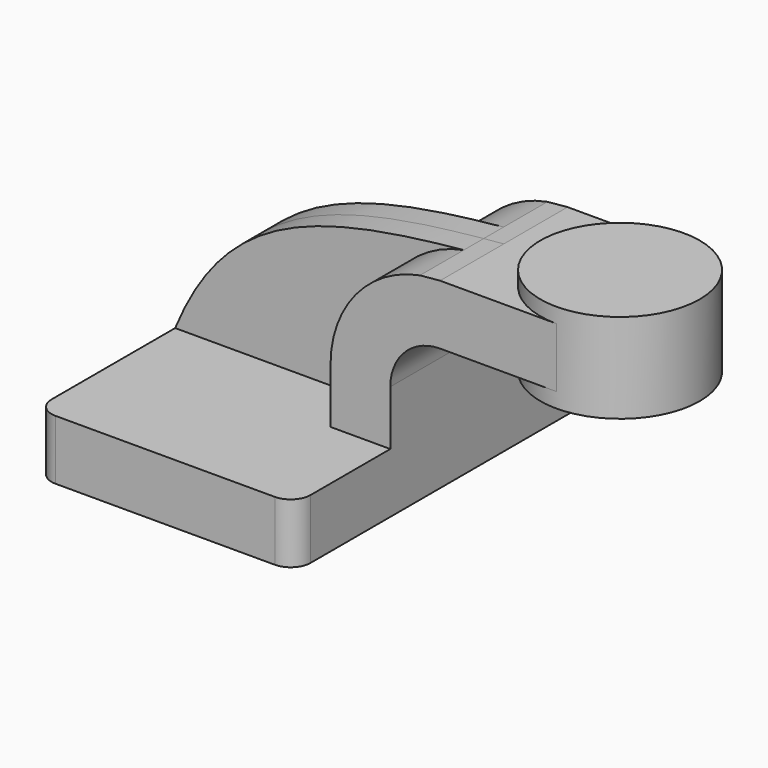
from build123d import *

# Parameters (mm, degrees)
F1_DEPTH = 63.5
F2_DEPTH = 25.4
F3_DEPTH = 7.9375
F0_W     = 25.4
F0_H     = 19.05
F4_DEPTH = 25.4
F6_R     = 6.35


# Not quite as in the source:
# - ends of sketch curves that miss each other by under 0.0002 mm in the source are joined
# - a feature names something its author has since deleted; it is built from what else it names


with BuildPart() as f1:
    # F0 (on Front) → F1 (new body, symmetric)
    with BuildSketch(Plane.XZ):
        Polygon((41.275, -9.525), (41.275, 9.525), (22.225, 9.525), (-41.275, 9.525), (-41.275, -9.525), align=None)
    extrude(amount=F1_DEPTH, both=True)

    # F0 (on Front) → F2 (join, symmetric)
    with BuildSketch(Plane.XZ):
        with BuildLine():
            Line((22.225, 9.525), (41.275, 9.525))
            Line((41.275, 9.525), (41.275, 27.0002))
            ThreePointArc((41.275, 27.0002), (45.9246798487, 38.2255201513), (57.15, 42.8752))
            Line((57.15, 42.8752), (68.7916731741, 42.8752))
            Line((68.7916731741, 42.8752), (68.7916731741, 61.9252))
            Line((68.7916731741, 61.9252), (57.15, 61.9252))
            add(Edge.make_bspline(
                [(50.7252492869, 61.329171511), (52.8269652502, 61.534305037), (54.9682888804, 61.732284225), (57.15, 61.9252)],
                knots=[106.8911851376, 106.8911851376, 106.8911851376, 106.8911851376, 111.5045367133, 111.5045367133, 111.5045367133, 111.5045367133], degree=3))
            ThreePointArc((50.7252492869, 61.329171511), (30.2786385449, 49.3090690945), (22.22499883, 27.0002))
            Line((22.22499883, 27.0002), (22.225, 9.525))
        make_face()
    extrude(amount=F2_DEPTH, both=True)

    # F0 (on Front) → F3 (join, symmetric)
    with BuildSketch(Plane.XZ):
        with BuildLine():
            Line((-41.275, 9.525), (22.225, 9.525))
            Line((22.225, 9.525), (22.225, 27.0002))
            ThreePointArc((22.225, 27.0002), (30.2786385449, 49.3090690945), (50.7252492869, 61.329171511))
            add(Edge.make_bspline(
                [(-41.275, 9.525), (-25.4048483065, 47.9825129098), (2.0285682627, 56.5762353117), (50.7252492869, 61.329171511)],
                knots=[0, 0, 0, 0, 106.8911851376, 106.8911851376, 106.8911851376, 106.8911851376], degree=3))
        make_face()
    extrude(amount=F3_DEPTH, both=True)

    # F0 (on Front) → F4 (join, symmetric)
    with BuildSketch(Plane.XZ):
        with Locations((81.4916731741, 52.4002)):
            Rectangle(F0_W, F0_H)
    extrude(amount=F4_DEPTH, both=True)

    # F0 (on Front) → F5 (revolve)
    with BuildSketch(Plane.XZ):
        Polygon((94.1916731741, 61.9252), (94.1916731741, 42.8752), (94.1916731741, 38.1), (119.5916731741, 38.1), (119.5916731741, 66.675), (94.1916731741, 66.675), align=None)
    revolve(axis=Axis((94.1916731741, 0, 52.3875), (0, 0, 1)))

    # F6
    f6_edges = [f1.edges().sort_by_distance(p)[0] for p in [
        (41.275, -63.5, 0),
        (-41.275, -63.5, 0),
        (41.275, 63.5, 0),
        (-41.275, 63.5, 0),
    ]]
    fillet(f6_edges, radius=F6_R)


solid = f1.part
